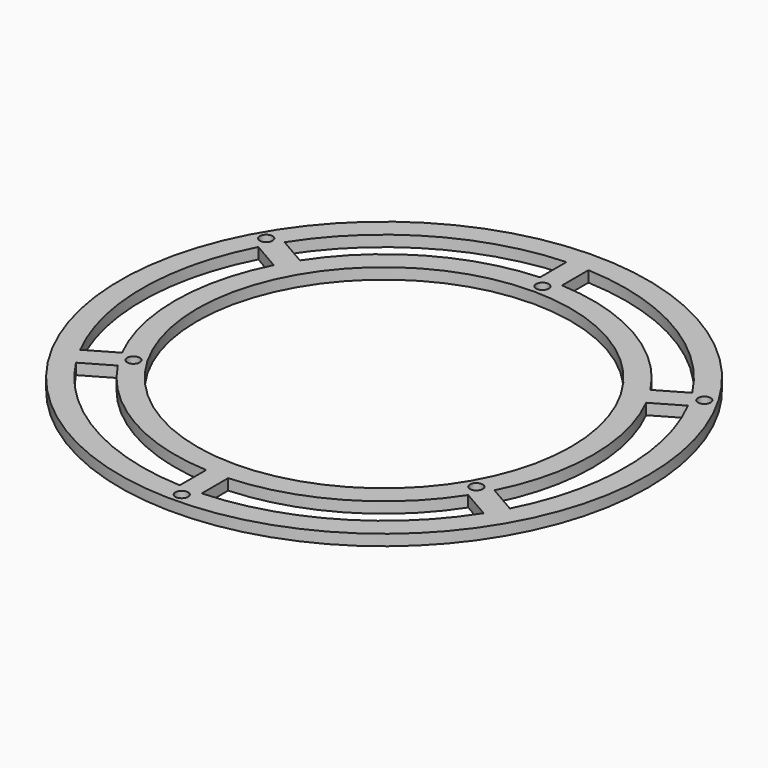
from build123d import *

# Parameters (mm, degrees)
F0_R            = 76.2
F0_R_2          = 1.8288
F0_R_3          = 53.975
F1_DEPTH        = 3.175
F3_DEPTH        = 3.175
F3_COPIES_COUNT = 6


# Not quite as in the source:
# - a pattern or mirror of a feature is missing from the dataset's text; its kind, count and spacing are read off the source's solid


with BuildPart() as f1:
    # F0 (on Top) → F1 (new body)
    with BuildSketch(Plane.XY):
        Circle(F0_R)
        with Locations((-49.4933518263, -28.575)):
            Circle(F0_R_2, mode=Mode.SUBTRACT)
        with Locations((0, -73.025)):
            Circle(F0_R_2, mode=Mode.SUBTRACT)
        with Locations((49.4933518263, -28.575)):
            Circle(F0_R_2, mode=Mode.SUBTRACT)
        with Locations((-63.2415051114, 36.5125)):
            Circle(F0_R_2, mode=Mode.SUBTRACT)
        Circle(F0_R_3, mode=Mode.SUBTRACT)
        with Locations((63.2415051114, 36.5125)):
            Circle(F0_R_2, mode=Mode.SUBTRACT)
        with Locations((0, 57.15)):
            Circle(F0_R_2, mode=Mode.SUBTRACT)
    extrude(amount=F1_DEPTH)

    # F2 (on face) → F3 (cut, through all)
    with BuildSketch(Plane.XY.offset(3.175)):
        with BuildLine():
            Line((-3.175, 60.2413894262), (-3.175, 69.7778035983))
            ThreePointArc((-3.175, 69.7778035983), (-34.925, 60.4918744543), (-58.8418505364, 37.6385324562))
            Line((-58.8418505364, 37.6385324562), (-50.5830736024, 32.8703253701))
            ThreePointArc((-50.5830736024, 32.8703253701), (-30.1625, 52.2429824833), (-3.175, 60.2413894262))
        make_face()
    f3 = extrude(amount=-F3_DEPTH, mode=Mode.SUBTRACT)

    # F3_copies: F3 ×6 about axis
    f3_copies_axis = Axis((0, 0, 0), (0, 0, 1))
    for i in range(1, F3_COPIES_COUNT):
        add(f3.rotate(f3_copies_axis, i * 360 / F3_COPIES_COUNT), mode=Mode.SUBTRACT)


solid = f1.part
